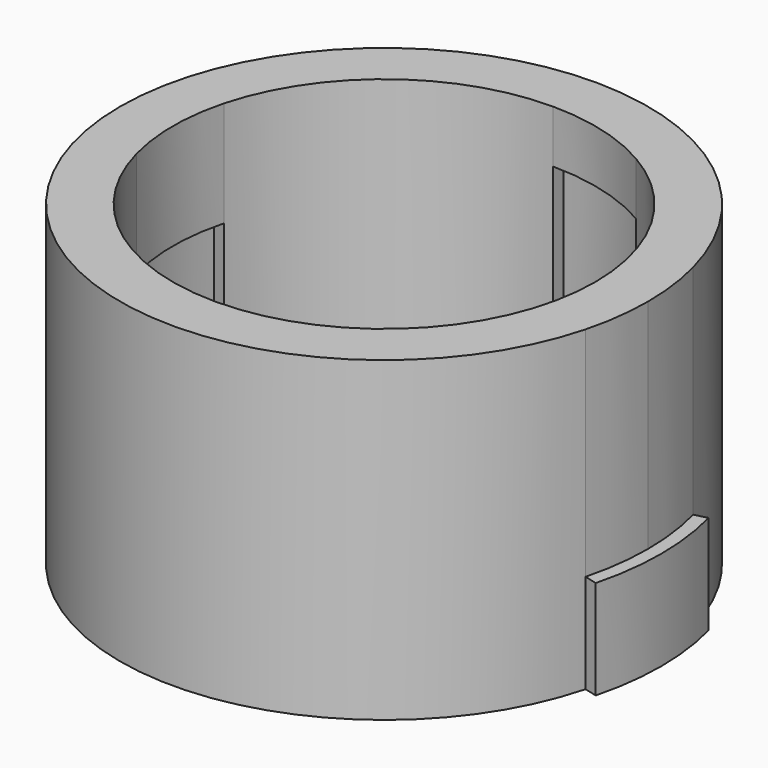
from build123d import *

# Parameters (mm, degrees)
F1_DEPTH = 76.2
F2_DEPTH = 23.8125
F3_DEPTH = 50.8
F4_DEPTH = 63.5
F5_DEPTH = 25.4


# Not quite as in the source:
# - a feature names something its author has since deleted; it is built from what else it names


with BuildPart() as f1:
    # F0 (on Top) → F1 (new body)
    with BuildSketch(Plane.XY):
        with BuildLine():
            ThreePointArc((61.4074185531, -16.1672182717), (62.9746817305, -8.151040482), (63.5, 0))
            ThreePointArc((63.5, 0), (62.9746817305, 8.151040482), (61.4074185531, 16.1672182717))
            ThreePointArc((61.4074185531, 16.1672182717), (0, 63.5), (-61.4074185531, 16.1672182717))
            ThreePointArc((-61.4074185531, 16.1672182717), (-63.5, 0), (-61.4074185531, -16.1672182717))
            ThreePointArc((-61.4074185531, -16.1672182717), (0, -63.5), (61.4074185531, -16.1672182717))
        make_face()
        with BuildLine():
            ThreePointArc((26.9875, 46.7437211693), (42.8212465422, 32.8578981307), (52.135846474, 13.9697579594))
            ThreePointArc((52.135846474, 13.9697579594), (53.5132363927, 7.0451512251), (53.975, 0))
            ThreePointArc((53.975, 0), (53.5132363927, -7.0451512251), (52.135846474, -13.9697579594))
            ThreePointArc((52.135846474, -13.9697579594), (32.8578981307, -42.8212465422), (0, -53.975))
            ThreePointArc((0, -53.975), (-13.9697579594, -52.135846474), (-26.9875, -46.7437211693))
            ThreePointArc((-26.9875, -46.7437211693), (-42.8212465422, -32.8578981307), (-52.135846474, -13.9697579594))
            ThreePointArc((-52.135846474, -13.9697579594), (-53.975, 0), (-52.135846474, 13.9697579594))
            ThreePointArc((-52.135846474, 13.9697579594), (-32.8578981307, 42.8212465422), (0, 53.975))
            ThreePointArc((0, 53.975), (13.9697579594, 52.135846474), (26.9875, 46.7437211693))
        make_face(mode=Mode.SUBTRACT)
        with BuildLine():
            ThreePointArc((49.0690319755, 13.1480074912), (50.3653989578, 6.6307305648), (50.8, 0))
            ThreePointArc((50.8, 0), (50.3653989578, -6.6307305648), (49.0690319755, -13.1480074912))
            Line((49.0690319755, -13.1480074912), (52.135846474, -13.9697579594))
            ThreePointArc((52.135846474, -13.9697579594), (53.5132363927, -7.0451512251), (53.975, 0))
            ThreePointArc((53.975, 0), (53.5132363927, 7.0451512251), (52.135846474, 13.9697579594))
            Line((52.135846474, 13.9697579594), (49.0690319755, 13.1480074912))
        make_face()
        with BuildLine():
            ThreePointArc((25.4, 43.9940905122), (40.3023496868, 30.9250805936), (49.0690319755, 13.1480074912))
            Line((49.0690319755, 13.1480074912), (52.135846474, 13.9697579594))
            ThreePointArc((52.135846474, 13.9697579594), (42.8212465422, 32.8578981307), (26.9875, 46.7437211693))
            Line((26.9875, 46.7437211693), (25.4, 43.9940905122))
        make_face()
        with BuildLine():
            Line((52.135846474, -13.9697579594), (49.0690319755, -13.1480074912))
            ThreePointArc((49.0690319755, -13.1480074912), (30.9250805936, -40.3023496868), (0, -50.8))
            Line((0, -50.8), (0, -53.975))
            ThreePointArc((0, -53.975), (32.8578981307, -42.8212465422), (52.135846474, -13.9697579594))
        make_face()
        with BuildLine():
            ThreePointArc((0, 50.8), (13.1480074912, 49.0690319755), (25.4, 43.9940905122))
            Line((25.4, 43.9940905122), (26.9875, 46.7437211693))
            ThreePointArc((26.9875, 46.7437211693), (13.9697579594, 52.135846474), (0, 53.975))
            Line((0, 53.975), (0, 50.8))
        make_face()
        with BuildLine():
            Line((0, -53.975), (0, -50.8))
            ThreePointArc((0, -50.8), (-13.1480074912, -49.0690319755), (-25.4, -43.9940905122))
            Line((-25.4, -43.9940905122), (-26.9875, -46.7437211693))
            ThreePointArc((-26.9875, -46.7437211693), (-13.9697579594, -52.135846474), (0, -53.975))
        make_face()
        with BuildLine():
            ThreePointArc((-49.0690319755, 13.1480074912), (-30.9250805936, 40.3023496868), (0, 50.8))
            Line((0, 50.8), (0, 53.975))
            ThreePointArc((0, 53.975), (-32.8578981307, 42.8212465422), (-52.135846474, 13.9697579594))
            Line((-52.135846474, 13.9697579594), (-49.0690319755, 13.1480074912))
        make_face()
        with BuildLine():
            Line((-26.9875, -46.7437211693), (-25.4, -43.9940905122))
            ThreePointArc((-25.4, -43.9940905122), (-40.3023496868, -30.9250805936), (-49.0690319755, -13.1480074912))
            Line((-49.0690319755, -13.1480074912), (-52.135846474, -13.9697579594))
            ThreePointArc((-52.135846474, -13.9697579594), (-42.8212465422, -32.8578981307), (-26.9875, -46.7437211693))
        make_face()
        with BuildLine():
            ThreePointArc((-49.0690319755, -13.1480074912), (-50.8, 0), (-49.0690319755, 13.1480074912))
            Line((-49.0690319755, 13.1480074912), (-52.135846474, 13.9697579594))
            ThreePointArc((-52.135846474, 13.9697579594), (-53.975, 0), (-52.135846474, -13.9697579594))
            Line((-52.135846474, -13.9697579594), (-49.0690319755, -13.1480074912))
        make_face()
    extrude(amount=F1_DEPTH)

    # F0 (on Top) → F2 (join)
    with BuildSketch(Plane.XY):
        with BuildLine():
            ThreePointArc((-61.4074185531, -16.1672182717), (-63.5, 0), (-61.4074185531, 16.1672182717))
            Line((-61.4074185531, 16.1672182717), (-64.4777894091, 16.9755794573))
            ThreePointArc((-64.4777894091, 16.9755794573), (-66.675, 0), (-64.4777894091, -16.9755794573))
            Line((-64.4777894091, -16.9755794573), (-61.4074185531, -16.1672182717))
        make_face()
        with BuildLine():
            ThreePointArc((61.4074185531, 16.1672182717), (62.9746817305, 8.151040482), (63.5, 0))
            ThreePointArc((63.5, 0), (62.9746817305, -8.151040482), (61.4074185531, -16.1672182717))
            Line((61.4074185531, -16.1672182717), (64.4777894091, -16.9755794573))
            ThreePointArc((64.4777894091, -16.9755794573), (66.675, 0), (64.4777894091, 16.9755794573))
            Line((64.4777894091, 16.9755794573), (61.4074185531, 16.1672182717))
        make_face()
    extrude(amount=F2_DEPTH)

    # F0 (on Top) → F3 (cut)
    with BuildSketch(Plane.XY):
        with BuildLine():
            ThreePointArc((-49.0690319755, -13.1480074912), (-50.8, 0), (-49.0690319755, 13.1480074912))
            Line((-49.0690319755, 13.1480074912), (-52.135846474, 13.9697579594))
            ThreePointArc((-52.135846474, 13.9697579594), (-53.975, 0), (-52.135846474, -13.9697579594))
            Line((-52.135846474, -13.9697579594), (-49.0690319755, -13.1480074912))
        make_face()
        with BuildLine():
            ThreePointArc((49.0690319755, 13.1480074912), (50.3653989578, 6.6307305648), (50.8, 0))
            ThreePointArc((50.8, 0), (50.3653989578, -6.6307305648), (49.0690319755, -13.1480074912))
            Line((49.0690319755, -13.1480074912), (52.135846474, -13.9697579594))
            ThreePointArc((52.135846474, -13.9697579594), (53.5132363927, -7.0451512251), (53.975, 0))
            ThreePointArc((53.975, 0), (53.5132363927, 7.0451512251), (52.135846474, 13.9697579594))
            Line((52.135846474, 13.9697579594), (49.0690319755, 13.1480074912))
        make_face()
        with BuildLine():
            Line((-26.9875, -46.7437211693), (-25.4, -43.9940905122))
            ThreePointArc((-25.4, -43.9940905122), (-40.3023496868, -30.9250805936), (-49.0690319755, -13.1480074912))
            Line((-49.0690319755, -13.1480074912), (-52.135846474, -13.9697579594))
            ThreePointArc((-52.135846474, -13.9697579594), (-42.8212465422, -32.8578981307), (-26.9875, -46.7437211693))
        make_face()
        with BuildLine():
            ThreePointArc((25.4, 43.9940905122), (40.3023496868, 30.9250805936), (49.0690319755, 13.1480074912))
            Line((49.0690319755, 13.1480074912), (52.135846474, 13.9697579594))
            ThreePointArc((52.135846474, 13.9697579594), (42.8212465422, 32.8578981307), (26.9875, 46.7437211693))
            Line((26.9875, 46.7437211693), (25.4, 43.9940905122))
        make_face()
    extrude(amount=F3_DEPTH, mode=Mode.SUBTRACT)

    # F0 (on Top) → F4 (cut)
    with BuildSketch(Plane.XY):
        with BuildLine():
            Line((0, -53.975), (0, -50.8))
            ThreePointArc((0, -50.8), (-13.1480074912, -49.0690319755), (-25.4, -43.9940905122))
            Line((-25.4, -43.9940905122), (-26.9875, -46.7437211693))
            ThreePointArc((-26.9875, -46.7437211693), (-13.9697579594, -52.135846474), (0, -53.975))
        make_face()
        with BuildLine():
            ThreePointArc((0, 50.8), (13.1480074912, 49.0690319755), (25.4, 43.9940905122))
            Line((25.4, 43.9940905122), (26.9875, 46.7437211693))
            ThreePointArc((26.9875, 46.7437211693), (13.9697579594, 52.135846474), (0, 53.975))
            Line((0, 53.975), (0, 50.8))
        make_face()
    extrude(amount=F4_DEPTH, mode=Mode.SUBTRACT)

    # F0 (on Top) → F5 (join)
    with BuildSketch(Plane.XY):
        with BuildLine():
            Line((-26.9875, -46.7437211693), (-25.4, -43.9940905122))
            ThreePointArc((-25.4, -43.9940905122), (-40.3023496868, -30.9250805936), (-49.0690319755, -13.1480074912))
            Line((-49.0690319755, -13.1480074912), (-52.135846474, -13.9697579594))
            ThreePointArc((-52.135846474, -13.9697579594), (-42.8212465422, -32.8578981307), (-26.9875, -46.7437211693))
        make_face()
        with BuildLine():
            Line((0, -53.975), (0, -50.8))
            ThreePointArc((0, -50.8), (-13.1480074912, -49.0690319755), (-25.4, -43.9940905122))
            Line((-25.4, -43.9940905122), (-26.9875, -46.7437211693))
            ThreePointArc((-26.9875, -46.7437211693), (-13.9697579594, -52.135846474), (0, -53.975))
        make_face()
        with BuildLine():
            ThreePointArc((25.4, 43.9940905122), (40.3023496868, 30.9250805936), (49.0690319755, 13.1480074912))
            Line((49.0690319755, 13.1480074912), (52.135846474, 13.9697579594))
            ThreePointArc((52.135846474, 13.9697579594), (42.8212465422, 32.8578981307), (26.9875, 46.7437211693))
            Line((26.9875, 46.7437211693), (25.4, 43.9940905122))
        make_face()
        with BuildLine():
            ThreePointArc((0, 50.8), (13.1480074912, 49.0690319755), (25.4, 43.9940905122))
            Line((25.4, 43.9940905122), (26.9875, 46.7437211693))
            ThreePointArc((26.9875, 46.7437211693), (13.9697579594, 52.135846474), (0, 53.975))
            Line((0, 53.975), (0, 50.8))
        make_face()
    extrude(amount=F5_DEPTH)


solid = f1.part
